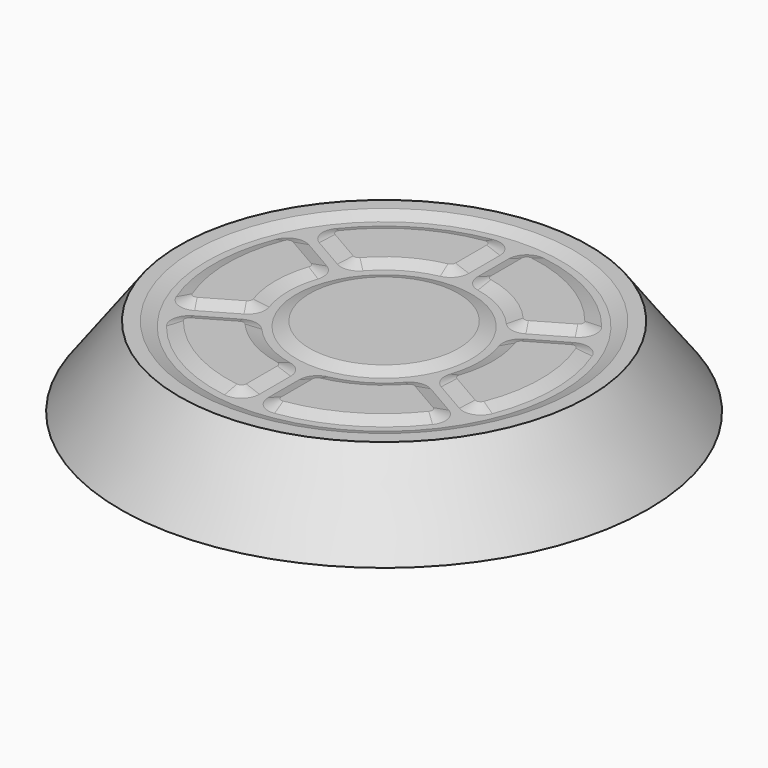
from build123d import *

# Parameters (mm, degrees)
F0_R                   = 64
F2_R                   = 82.5
F5_DEPTH               = 1.5
DRAFT_F5_DRAFTED_ANGLE = 70
F6_T                   = -0.5


# Not quite as in the source:
# - an extrude with a draft is written as a straight extrude whose walls are then drafted


with BuildPart() as f3:
    # F0 (on Top) → F3 section 0
    with BuildSketch(Plane.XY):
        Circle(F0_R)
    # F2 (on offset) → F3 section 1
    with BuildSketch(Plane.XY.offset(-25)):
        Circle(F2_R)
    loft()


with BuildPart() as f5_drafted:
    # F4 (on face) → F5 (new body)
    with BuildSketch(Plane.XY):
        with BuildLine():
            ThreePointArc((0, 59.5), (-42.0728534806, -42.0728534806), (59.5, 0))
            ThreePointArc((59.5, 0), (42.0728534806, 42.0728534806), (0, 59.5))
        make_face()
        with BuildLine():
            ThreePointArc((-7.2210526316, -48.465001794), (-24.5, -42.4352447854), (-38.3613964323, -30.486115918))
            ThreePointArc((-38.3613964323, -30.486115918), (-38.6606811555, -29.2727528885), (-37.9370679701, -28.2538293659))
            Line((-37.9370679701, -28.2538293659), (-27.3902969461, -22.1646482761))
            ThreePointArc((-27.3902969461, -22.1646482761), (-26.3975331685, -21.9834614839), (-25.5146505963, -22.4722630135))
            ThreePointArc((-25.5146505963, -22.4722630135), (-17, -29.4448637287), (-6.7042253521, -33.3324670918))
            ThreePointArc((-6.7042253521, -33.3324670918), (-5.8394695239, -33.8526650631), (-5.5, -34.8030171106))
            Line((-5.5, -34.8030171106), (-5.5, -46.9813792901))
            ThreePointArc((-5.5, -46.9813792901), (-6.0206070624, -48.1175084525), (-7.2210526316, -48.465001794))
        make_face(mode=Mode.SUBTRACT)
        with BuildLine():
            ThreePointArc((38.3613964323, -30.486115918), (24.5, -42.4352447854), (7.2210526316, -48.465001794))
            ThreePointArc((7.2210526316, -48.465001794), (6.0206070624, -48.1175084525), (5.5, -46.9813792901))
            Line((5.5, -46.9813792901), (5.5, -34.8030171106))
            ThreePointArc((5.5, -34.8030171106), (5.8394695239, -33.8526650631), (6.7042253521, -33.3324670918))
            ThreePointArc((6.7042253521, -33.3324670918), (17, -29.4448637287), (25.5146505963, -22.4722630135))
            ThreePointArc((25.5146505963, -22.4722630135), (26.3975331685, -21.9834614839), (27.3902969461, -22.1646482761))
            Line((27.3902969461, -22.1646482761), (37.9370679701, -28.2538293659))
            ThreePointArc((37.9370679701, -28.2538293659), (38.6606811555, -29.2727528885), (38.3613964323, -30.486115918))
        make_face(mode=Mode.SUBTRACT)
        with BuildLine():
            ThreePointArc((45.5824490638, 17.978885876), (49, 0), (45.5824490638, -17.978885876))
            ThreePointArc((45.5824490638, -17.978885876), (44.6812882179, -18.8447555641), (43.4370679701, -18.7275499242))
            Line((43.4370679701, -18.7275499242), (32.8902969461, -12.6383688345))
            ThreePointArc((32.8902969461, -12.6383688345), (32.2370026924, -11.8692035792), (32.2188759484, -10.8602040783))
            ThreePointArc((32.2188759484, -10.8602040783), (34, 0), (32.2188759484, 10.8602040783))
            ThreePointArc((32.2188759484, 10.8602040783), (32.2370026924, 11.8692035792), (32.8902969461, 12.6383688345))
            Line((32.8902969461, 12.6383688345), (43.4370679701, 18.7275499242))
            ThreePointArc((43.4370679701, 18.7275499242), (44.6812882179, 18.8447555641), (45.5824490638, 17.978885876))
        make_face(mode=Mode.SUBTRACT)
        with BuildLine():
            ThreePointArc((-45.5824490638, -17.978885876), (-49, 0), (-45.5824490638, 17.978885876))
            ThreePointArc((-45.5824490638, 17.978885876), (-44.6812882179, 18.8447555641), (-43.4370679701, 18.7275499242))
            Line((-43.4370679701, 18.7275499242), (-32.8902969461, 12.6383688345))
            ThreePointArc((-32.8902969461, 12.6383688345), (-32.2370026924, 11.8692035792), (-32.2188759484, 10.8602040783))
            ThreePointArc((-32.2188759484, 10.8602040783), (-34, 0), (-32.2188759484, -10.8602040783))
            ThreePointArc((-32.2188759484, -10.8602040783), (-32.2370026924, -11.8692035792), (-32.8902969461, -12.6383688345))
            Line((-32.8902969461, -12.6383688345), (-43.4370679701, -18.7275499242))
            ThreePointArc((-43.4370679701, -18.7275499242), (-44.6812882179, -18.8447555641), (-45.5824490638, -17.978885876))
        make_face(mode=Mode.SUBTRACT)
        with BuildLine():
            ThreePointArc((-38.3613964323, 30.486115918), (-24.5, 42.4352447854), (-7.2210526316, 48.465001794))
            ThreePointArc((-7.2210526316, 48.465001794), (-6.0206070624, 48.1175084525), (-5.5, 46.9813792901))
            Line((-5.5, 46.9813792901), (-5.5, 34.8030171106))
            ThreePointArc((-5.5, 34.8030171106), (-5.8394695239, 33.8526650631), (-6.7042253521, 33.3324670918))
            ThreePointArc((-6.7042253521, 33.3324670918), (-17, 29.4448637287), (-25.5146505963, 22.4722630135))
            ThreePointArc((-25.5146505963, 22.4722630135), (-26.3975331685, 21.9834614839), (-27.3902969461, 22.1646482761))
            Line((-27.3902969461, 22.1646482761), (-37.9370679701, 28.2538293659))
            ThreePointArc((-37.9370679701, 28.2538293659), (-38.6606811555, 29.2727528885), (-38.3613964323, 30.486115918))
        make_face(mode=Mode.SUBTRACT)
        with BuildLine():
            ThreePointArc((-20.135090638, 11.625), (-11.625, 20.135090638), (0, 23.25))
            ThreePointArc((0, 23.25), (16.4402326626, 16.4402326626), (23.25, 0))
            ThreePointArc((23.25, 0), (-6.0175427986, -22.4577754612), (-20.135090638, 11.625))
        make_face(mode=Mode.SUBTRACT)
        with BuildLine():
            ThreePointArc((7.2210526316, 48.465001794), (24.5, 42.4352447854), (38.3613964323, 30.486115918))
            ThreePointArc((38.3613964323, 30.486115918), (38.6606811555, 29.2727528885), (37.9370679701, 28.2538293659))
            Line((37.9370679701, 28.2538293659), (27.3902969461, 22.1646482761))
            ThreePointArc((27.3902969461, 22.1646482761), (26.3975331685, 21.9834614839), (25.5146505963, 22.4722630135))
            ThreePointArc((25.5146505963, 22.4722630135), (17, 29.4448637287), (6.7042253521, 33.3324670918))
            ThreePointArc((6.7042253521, 33.3324670918), (5.8394695239, 33.8526650631), (5.5, 34.8030171106))
            Line((5.5, 34.8030171106), (5.5, 46.9813792901))
            ThreePointArc((5.5, 46.9813792901), (6.0206070624, 48.1175084525), (7.2210526316, 48.465001794))
        make_face(mode=Mode.SUBTRACT)
    extrude(amount=-F5_DEPTH)

    # draft_F5_drafted
    draft_f5_drafted_walls = [f5_drafted.faces().sort_by_distance(p)[0] for p in [
        (-59.5, 0, -1),
        (6.0206070624, 48.1175084525, -1),
        (5.5, 40.8921982003, -1),
        (5.8394695239, 33.8526650631, -1),
        (17, 29.4448637287, -1),
        (26.3975331685, 21.9834614839, -1),
        (32.6636824581, 25.209238821, -1),
        (38.6606811555, 29.2727528885, -1),
        (24.5, 42.4352447854, -1),
        (20.135090638, -11.625, -1),
        (-38.6606811555, 29.2727528885, -1),
        (-32.6636824581, 25.209238821, -1),
        (-26.3975331685, 21.9834614839, -1),
        (-17, 29.4448637287, -1),
        (-5.8394695239, 33.8526650631, -1),
        (-5.5, 40.8921982003, -1),
        (-6.0206070624, 48.1175084525, -1),
        (-24.5, 42.4352447854, -1),
        (-44.6812882179, -18.8447555641, -1),
        (-38.1636824581, -15.6829593794, -1),
        (-32.2370026924, -11.8692035792, -1),
        (-34, 0, -1),
        (-32.2370026924, 11.8692035792, -1),
        (-38.1636824581, 15.6829593794, -1),
        (-44.6812882179, 18.8447555641, -1),
        (-49, 0, -1),
        (44.6812882179, 18.8447555641, -1),
        (38.1636824581, 15.6829593794, -1),
        (32.2370026924, 11.8692035792, -1),
        (34, 0, -1),
        (32.2370026924, -11.8692035792, -1),
        (38.1636824581, -15.6829593794, -1),
        (44.6812882179, -18.8447555641, -1),
        (49, 0, -1),
        (38.6606811555, -29.2727528885, -1),
        (32.6636824581, -25.209238821, -1),
        (26.3975331685, -21.9834614839, -1),
        (17, -29.4448637287, -1),
        (5.8394695239, -33.8526650631, -1),
        (5.5, -40.8921982003, -1),
        (6.0206070624, -48.1175084525, -1),
        (24.5, -42.4352447854, -1),
        (-6.0206070624, -48.1175084525, -1),
        (-5.5, -40.8921982003, -1),
        (-5.8394695239, -33.8526650631, -1),
        (-17, -29.4448637287, -1),
        (-26.3975331685, -21.9834614839, -1),
        (-32.6636824581, -25.209238821, -1),
        (-38.6606811555, -29.2727528885, -1),
        (-24.5, -42.4352447854, -1),
    ]]
    draft(draft_f5_drafted_walls, neutral_plane=Plane(origin=(0, 0, 0), x_dir=(1, 0, 0), z_dir=(0, 0, -1)), angle=DRAFT_F5_DRAFTED_ANGLE)


with BuildPart() as f3_1:
    add(f3.part)

    # join_F5_drafted: cut F5_drafted
    add(f5_drafted.part, mode=Mode.SUBTRACT)

    # F6
    f6_openings = [f3_1.faces().sort_by_distance(p)[0] for p in [
        (0, 0, -25),
    ]]
    offset(amount=F6_T, openings=f6_openings, kind=Kind.INTERSECTION)


solid = f3_1.part
